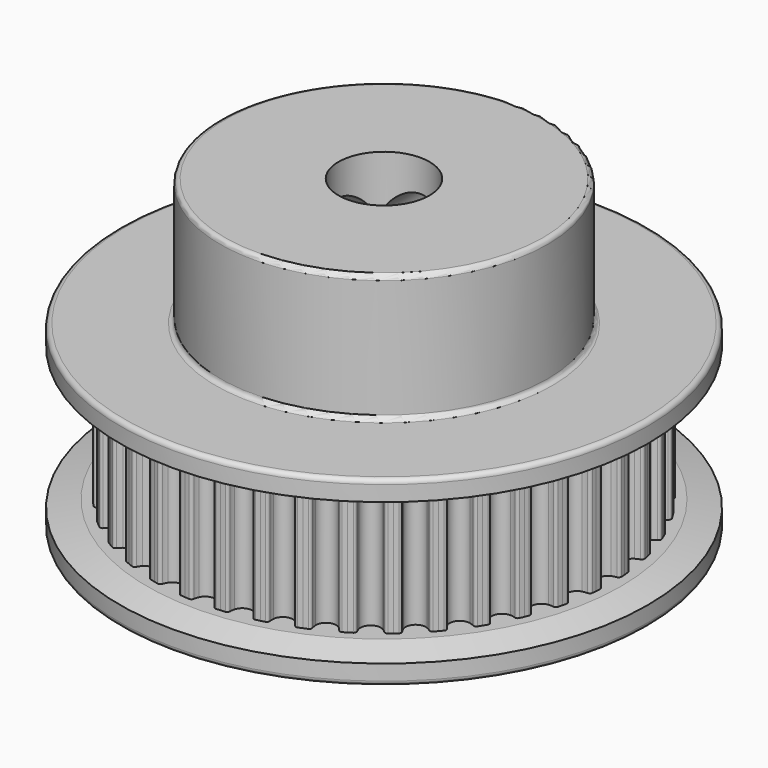
from build123d import *

# Parameters (mm, degrees)
F3_DEPTH    = 3.5
F4_COUNT    = 40
F5_R        = 14.5
F6_DEPTH    = 1.5
F7_R        = 14.5
F8_DEPTH    = 1.5
F9_R        = 9
F10_DEPTH   = 7
F11_R       = 2.5
F12_DEPTH   = 17.001
F13_R       = 1.75
F14_DEPTH   = 14.501
F15_R       = 1.75
F16_DEPTH   = 14.501
F17_SIZE2   = 0.4019237886
F17_SIZE    = 1.5
F17_2_SIZE2 = 0.4019237886
F17_2_SIZE  = 1.5
F18_R       = 0.25


# Not quite as in the source:
# - a feature names something its author has since deleted; it is built from what else it names


with BuildPart() as f3:
    # F2 (on Top) → F3 (new body, symmetric)
    with BuildSketch(Plane.XY):
        with BuildLine():
            ThreePointArc((0.5075167453, 12.0670474738), (0.3027902361, 11.8265352082), (0, 11.736662151))
            ThreePointArc((0, 11.736662151), (-0.3027902361, 11.8265352082), (-0.5075167453, 12.0670474738))
            ThreePointArc((-0.5075167453, 12.0670474738), (-0.5540316074, 12.1950693578), (-0.5827175627, 12.3282247224))
            ThreePointArc((-0.5827175627, 12.3282247224), (-0.6364131874, 12.4229796898), (-0.7400604747, 12.4564306057))
            ThreePointArc((-0.7400604747, 12.4564306057), (-0.8595916488, 12.448753156), (-0.9790436229, 12.4399287186))
            Line((-0.9790436229, 12.4399287186), (0, 0))
            Line((0, 0), (0.9790436229, 12.4399287186))
            ThreePointArc((0.9790436229, 12.4399287186), (0.8595916488, 12.448753156), (0.7400604747, 12.4564306057))
            ThreePointArc((0.7400604747, 12.4564306057), (0.6364131874, 12.4229796898), (0.5827175627, 12.3282247224))
            ThreePointArc((0.5827175627, 12.3282247224), (0.5540316074, 12.1950693578), (0.5075167453, 12.0670474738))
        make_face()
    extrude(amount=F3_DEPTH, both=True)

    # F4: F3 ×40 about axis
    f4_axis = Axis((0, 0, 0), (0, 0, -1))


with BuildPart() as f3_1:
    add(f3.part)
    for i in range(1, F4_COUNT):
        add(f3.part.rotate(f4_axis, i * 360 / F4_COUNT))

    # F5 (on face) → F6 (join)
    with BuildSketch(Plane(origin=(0, 0, -3.5), x_dir=(1, 0, 0), z_dir=(0, 0, -1))):
        Circle(F5_R)
    extrude(amount=F6_DEPTH)

    # F7 (on face) → F8 (join)
    with BuildSketch(Plane.XY.offset(3.5)):
        Circle(F7_R)
    extrude(amount=F8_DEPTH)

    # F9 (on face) → F10 (join)
    with BuildSketch(Plane.XY.offset(5)):
        Circle(F9_R)
    extrude(amount=F10_DEPTH)

    # F11 (on face) → F12 (cut, through all)
    with BuildSketch(Plane.XY.offset(12)):
        Circle(F11_R)
    extrude(amount=-F12_DEPTH, mode=Mode.SUBTRACT)

    # F13 (on Front) → F14 (cut, through all)
    with BuildSketch(Plane.XZ):
        with Locations((0, 8.5)):
            Circle(F13_R)
    extrude(amount=-F14_DEPTH, mode=Mode.SUBTRACT)

    # F15 (on Right) → F16 (cut, through all)
    with BuildSketch(Plane.YZ):
        with Locations((0, 8.5)):
            Circle(F15_R)
    extrude(amount=-F16_DEPTH, mode=Mode.SUBTRACT)

    # F17
    f17_edges = [f3_1.edges().sort_by_distance(p)[0] for p in [
        (-14.5, 0, -3.5),
    ]]
    f17_side = f3_1.faces().sort_by_distance((-14.089878, 0, -3.5))[0]
    chamfer(f17_edges, length=F17_SIZE, length2=F17_SIZE2, reference=f17_side)

    # F17#2
    f17_2_edges = [f3_1.edges().sort_by_distance(p)[0] for p in [
        (-14.5, 0, 3.5),
    ]]
    f17_2_side = f3_1.faces().sort_by_distance((-14.089878, 0, 3.5))[0]
    chamfer(f17_2_edges, length=F17_2_SIZE, length2=F17_2_SIZE2, reference=f17_2_side)

    # F18
    f18_edges = [f3_1.edges().sort_by_distance(p)[0] for p in [
        (-9, 0, 5),
        (-9, 0, 12),
        (-14.5, 0, 5),
        (-14.5, 0, -5),
    ]]
    fillet(f18_edges, radius=F18_R)


solid = f3_1.part
